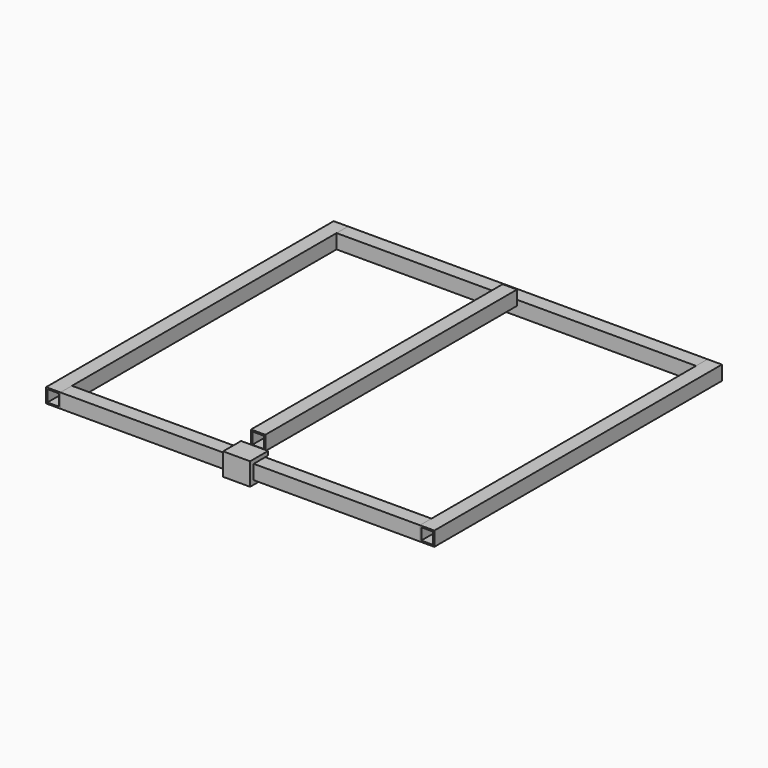
from build123d import *

# Parameters (mm, degrees)
F0_W          = 16
F0_H          = 16
F0_W_2        = 13
F0_H_2        = 13
F1_DEPTH      = 200
F2_W          = 16
F2_H          = 16
F2_W_2        = 13
F2_H_2        = 13
F3_DEPTH      = 200
F3_DEPTH_BACK = 200
F5_W          = 16
F5_H          = 16
F5_W_2        = 13
F5_H_2        = 13
F6_DEPTH      = 175
F7_W          = 30
F7_H          = 4.5
F8_DEPTH      = 20
F7_H_2        = 16
F9_DEPTH      = 5


with BuildPart() as f1:
    # F0 (on Front) → F1 (new body, symmetric)
    with BuildSketch(Plane.XZ):
        with Locations((-208, 0)):
            Rectangle(F0_W, F0_H)
        with Locations((-208, 0)):
            Rectangle(F0_W_2, F0_H_2, mode=Mode.SUBTRACT)
    extrude(amount=F1_DEPTH, both=True)


with BuildPart() as f1b:
    # F0 (on Front) → F1, piece 2 (new body, symmetric)
    with BuildSketch(Plane.XZ):
        with Locations((208, 0)):
            Rectangle(F0_W, F0_H)
        with Locations((208, 0)):
            Rectangle(F0_W_2, F0_H_2, mode=Mode.SUBTRACT)
    extrude(amount=F1_DEPTH, both=True)


with BuildPart() as f3:
    # F2 (on Right) → F3 (new body, two sides)
    with BuildSketch(Plane.YZ) as f3_sk:
        with Locations((-192, 0)):
            Rectangle(F2_W, F2_H)
        with Locations((-192, 0)):
            Rectangle(F2_W_2, F2_H_2, mode=Mode.SUBTRACT)
    extrude(amount=F3_DEPTH)
    extrude(f3_sk.sketch, amount=-F3_DEPTH_BACK)


with BuildPart() as f3b:
    # F2 (on Right) → F3, piece 2 (new body, two sides)
    with BuildSketch(Plane.YZ) as f3_2_sk:
        with Locations((192, 0)):
            Rectangle(F2_W, F2_H)
        with Locations((192, 0)):
            Rectangle(F2_W_2, F2_H_2, mode=Mode.SUBTRACT)
    extrude(amount=F3_DEPTH)
    extrude(f3_2_sk.sketch, amount=-F3_DEPTH_BACK)


with BuildPart() as f6:
    # F5 (on Front) → F6 (new body, symmetric)
    with BuildSketch(Plane.XZ):
        with Locations((2e-10, 16)):
            Rectangle(F5_W, F5_H)
        with Locations((2e-10, 16)):
            Rectangle(F5_W_2, F5_H_2, mode=Mode.SUBTRACT)
    extrude(amount=F6_DEPTH, both=True)


with BuildPart() as f8:
    # F7 (on face) → F8 (new body)
    with BuildSketch(Plane.XZ.offset(200)):
        with Locations((0, 10.25)):
            Rectangle(F7_W, F7_H)
    extrude(amount=-F8_DEPTH)



with BuildPart() as f8b:
    # F7 (on face) → F8, piece 2 (new body)
    with BuildSketch(Plane.XZ.offset(200)):
        with Locations((0, -10.25)):
            Rectangle(F7_W, F7_H)
    extrude(amount=-F8_DEPTH)


with BuildPart() as f8_1:
    add(f8.part)

    add(f8b.part)  # F9 merges F8b
    # F7 (on face) → F9 (join)
    with BuildSketch(Plane.XZ.offset(200)):
        with Locations((0, 10.25)):
            Rectangle(F7_W, F7_H)
        Rectangle(F7_W, F7_H_2)
        with Locations((0, -10.25)):
            Rectangle(F7_W, F7_H)
    extrude(amount=F9_DEPTH)


solid = Compound([f1.part, f1b.part, f3.part, f3b.part, f6.part, f8_1.part])
